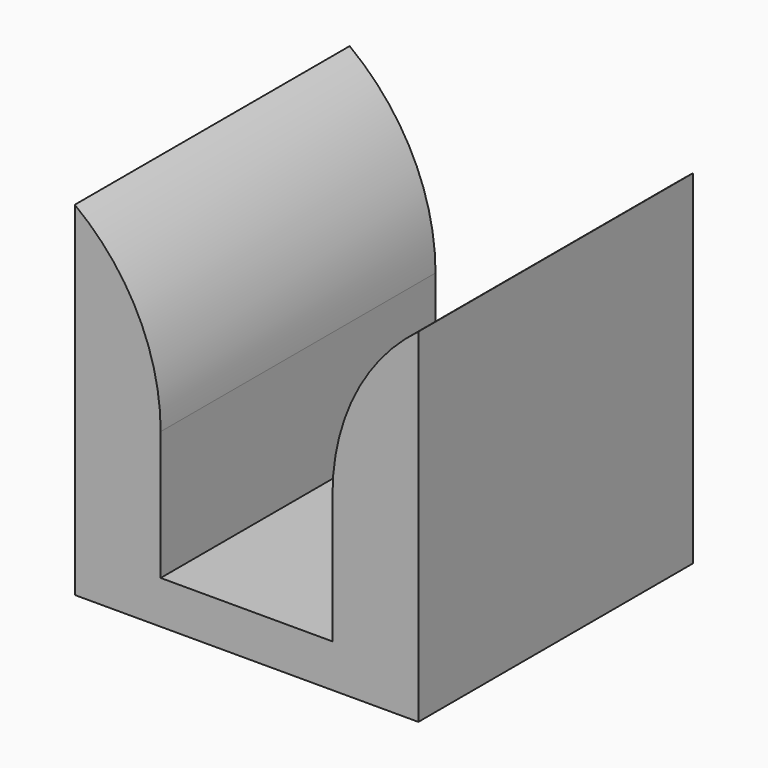
from build123d import *

# Parameters (mm, degrees)
F0_W        = 2
F0_H        = 7
F1_DEPTH    = 8
F2_T1_DEPTH = 28


# Not quite as in the source:
# - a fillet or chamfer that OpenCascade refuses, or shapes differently, is made with other operations: its cross-section is extruded or revolved along the edge and cut away or added


with BuildPart() as f1:
    # F0 (on Front) → F1 (new body)
    with BuildSketch(Plane.XZ):
        with Locations((-3, 4)):
            Rectangle(F0_W, F0_H)
        Polygon((-2, 0.5), (-4, 0.5), (-4, -0.5), (4, -0.5), (4, 0.5), (2, 0.5), align=None)
        with Locations((3, 4)):
            Rectangle(F0_W, F0_H)
    extrude(amount=F1_DEPTH)

    # F2: fillet of radius 5 on 2 edges, made by hand

    # F2_s2 → F2_t1 (cut)
    with BuildSketch(Plane.XZ.offset(-10)):
        with BuildLine():
            ThreePointArc((-2, 3.5), (-2.527864045, 5.7360679775), (-4, 7.5))
            Line((-4, 7.5), (-2, 7.5))
            Line((-2, 7.5), (-2, 3.5))
        make_face()
        with BuildLine():
            ThreePointArc((4, 7.5), (2.527864045, 5.7360679775), (2, 3.5))
            Line((2, 3.5), (2, 7.5))
            Line((2, 7.5), (4, 7.5))
        make_face()
    extrude(amount=F2_T1_DEPTH, mode=Mode.SUBTRACT)


solid = f1.part
